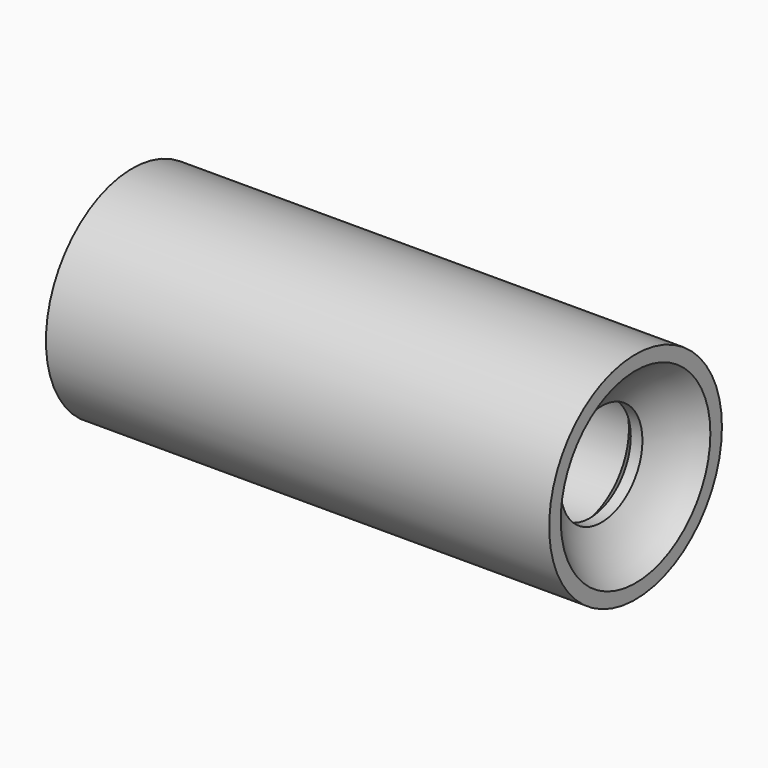
from build123d import *

# Parameters (mm, degrees)
F2_SIZE = 0.09999


# Not quite as in the source:
# - a fillet or chamfer is up to 0.001 mm smaller than in the source, because OpenCascade refuses the exact size


with BuildPart() as f1:
    # F0 (on Top) → F1 (revolve)
    with BuildSketch(Plane.XY):
        Polygon((6.425, 3.3), (6.925, 2.8), (6.925, 3.3), align=None)
        with BuildLine():
            ThreePointArc((7.5617104388, 2.8), (8.3591026496, 4.0638625595), (9.425, 5.1112620751))
            Line((9.425, 5.1112620751), (9.425, 5.9))
            Line((9.425, 5.9), (-18.075, 5.9))
            Line((-18.075, 5.9), (-18.075, 3.4))
            Line((-18.075, 3.4), (-7.075, 3.4))
            Line((-7.075, 3.4), (-7.075, 3.3))
            Line((-7.075, 3.3), (-6.425, 3.3))
            Line((-6.425, 3.3), (6.425, 3.3))
            Line((6.425, 3.3), (6.925, 3.3))
            Line((6.925, 3.3), (6.925, 2.8))
            Line((6.925, 2.8), (7.5617104388, 2.8))
        make_face()
    revolve(axis=Axis((1.3457932509, 0, 0), (1, 0, 0)))

    # F2 (size 0.1 in the source; OpenCascade refuses exactly that, so slightly less here)
    f2_edges = [f1.edges().sort_by_distance(p)[0] for p in [
        (-7.075, -3.4, 0),
    ]]
    chamfer(f2_edges, length=F2_SIZE)


solid = f1.part
